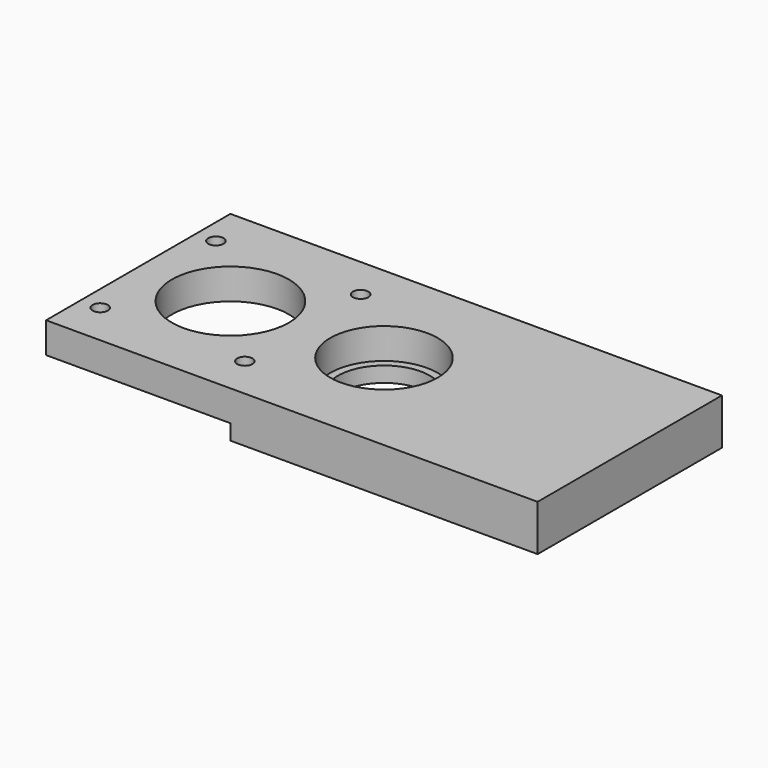
from build123d import *

# Parameters (mm, degrees)
F0_W     = 160
F0_H     = 75
F0_R     = 17.5
F1_DEPTH = 15
F2_R     = 2.5
F2_R_2   = 19.05
F3_DEPTH = 25
F4_R     = 4
F5_DEPTH = 11
F6_W     = 60
F6_H     = 5
F7_DEPTH = 79.7
F8_R     = 19
F8_R_2   = 17.5
F8_R_3   = 15
F9_DEPTH = 5


# Not quite as in the source:
# - a feature names something its author has since deleted; it is built from what else it names


with BuildPart() as f1:
    # F0 (on Top) → F1 (new body)
    with BuildSketch(Plane.XY):
        Rectangle(F0_W, F0_H)
        Circle(F0_R, mode=Mode.SUBTRACT)
    extrude(amount=F1_DEPTH)

    # F2 (on face) → F3 (cut)
    with BuildSketch(Plane.XY.offset(15)):
        with Locations((-73.55, 23.55)):
            Circle(F2_R)
        with Locations((-26.45, 23.55)):
            Circle(F2_R)
        with Locations((-26.45, -23.55)):
            Circle(F2_R)
        with Locations((-73.55, -23.55)):
            Circle(F2_R)
        with Locations((-50, 0)):
            Circle(F2_R_2)
    extrude(amount=-F3_DEPTH, mode=Mode.SUBTRACT)

    # F4 (on face) → F5 (cut)
    with BuildSketch(Plane(origin=(0, 0, 0), x_dir=(1, 0, 0), z_dir=(0, 0, -1))):
        with Locations((-73.55, 23.55)):
            Circle(F4_R)
        with Locations((-26.45, 23.55)):
            Circle(F4_R)
        with Locations((-26.45, -23.55)):
            Circle(F4_R)
        with Locations((-73.55, -23.55)):
            Circle(F4_R)
    extrude(amount=-F5_DEPTH, mode=Mode.SUBTRACT)

    # F6 (on face) → F7 (cut)
    with BuildSketch(Plane.XZ.offset(37.5)):
        with Locations((-50, 2.5)):
            Rectangle(F6_W, F6_H)
    extrude(amount=-F7_DEPTH, mode=Mode.SUBTRACT)

    # F8 (on face) → F9 (join)
    with BuildSketch(Plane(origin=(0, 0, 0), x_dir=(1, 0, 0), z_dir=(0, 0, -1))):
        Circle(F8_R)
        Circle(F8_R_2, mode=Mode.SUBTRACT)
        Circle(F8_R_2)
        Circle(F8_R_3, mode=Mode.SUBTRACT)
    extrude(amount=-F9_DEPTH)


solid = f1.part
